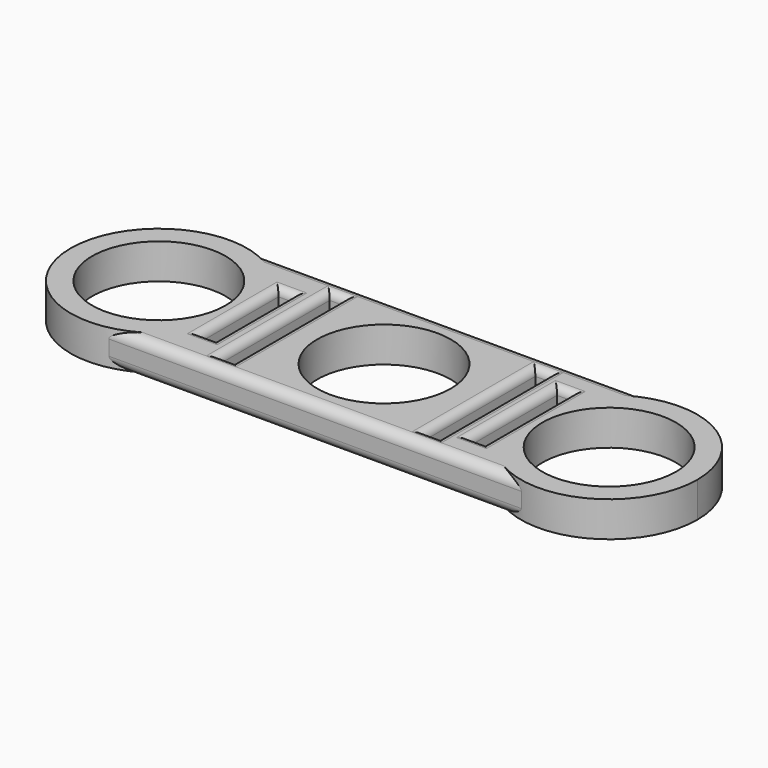
from build123d import *

# Parameters (mm, degrees)
F0_W          = 2.8743222356
F0_H          = 27.3038335145
F0_R          = 13.2535647779
F0_W_2        = 2.8743259609
F1_DEPTH      = 7
F2_R          = 2
F3_T1_DEPTH   = 19.2563887686
F3_T3_DEPTH   = 2.9194724291
F3_T5_DEPTH   = 27.3038335145
F3_T7_DEPTH   = 2.8743222356
F3_T9_DEPTH   = 2.8743259609
F3_T11_DEPTH  = 21.5556565672
F3_T13_DEPTH  = 2.9122043878
F3_T19_DEPTH  = 6.6694724291
F3_T23_DEPTH  = 23.0063887686
F3_T30_DEPTH  = 6.6694724291
F3_T34_DEPTH  = 23.0063887686
F3_T41_DEPTH  = 6.6694724291
F3_T45_DEPTH  = 23.0063887686
F3_T52_DEPTH  = 23.0063887686
F3_T56_DEPTH  = 6.6694724291
F3_T63_DEPTH  = 6.6243222356
F3_T67_DEPTH  = 31.0538335145
F3_T74_DEPTH  = 31.0538335145
F3_T78_DEPTH  = 6.6243222356
F3_T85_DEPTH  = 31.0538335145
F3_T89_DEPTH  = 6.6243222356
F3_T96_DEPTH  = 31.0538335145
F3_T100_DEPTH = 6.6243222356
F3_T107_DEPTH = 6.6243259609
F3_T111_DEPTH = 31.0538335145
F3_T118_DEPTH = 31.0538335145
F3_T122_DEPTH = 6.6243259609
F3_T129_DEPTH = 31.0538335145
F3_T133_DEPTH = 6.6243259609
F3_T140_DEPTH = 31.0538335145
F3_T144_DEPTH = 6.6243259609
F3_T151_DEPTH = 6.6622043878
F3_T155_DEPTH = 25.3056565672
F3_T162_DEPTH = 25.3056565672
F3_T166_DEPTH = 6.6622043878
F3_T173_DEPTH = 6.6622043878
F3_T177_DEPTH = 25.3056565672
F3_T184_DEPTH = 6.6622043878
F3_T188_DEPTH = 25.3056565672
F3_T195_DEPTH = 23.0063887686
F3_T199_DEPTH = 6.6694724291
F3_T206_DEPTH = 6.6694724291
F3_T210_DEPTH = 23.0063887686
F3_T217_DEPTH = 6.6694724291
F3_T221_DEPTH = 23.0063887686
F3_T228_DEPTH = 6.6694724291
F3_T232_DEPTH = 23.0063887686
F3_T239_DEPTH = 31.0538335145
F3_T243_DEPTH = 6.6243222356
F3_T250_DEPTH = 31.0538335145
F3_T254_DEPTH = 6.6243222356
F3_T261_DEPTH = 6.6243222356
F3_T265_DEPTH = 31.0538335145
F3_T272_DEPTH = 31.0538335145
F3_T276_DEPTH = 6.6243222356
F3_T283_DEPTH = 6.6243259609
F3_T287_DEPTH = 31.0538335145
F3_T294_DEPTH = 31.0538335145
F3_T298_DEPTH = 6.6243259609
F3_T305_DEPTH = 31.0538335145
F3_T309_DEPTH = 6.6243259609
F3_T316_DEPTH = 31.0538335145
F3_T320_DEPTH = 6.6243259609
F3_T327_DEPTH = 6.6622043878
F3_T331_DEPTH = 25.3056565672
F3_T338_DEPTH = 6.6622043878
F3_T342_DEPTH = 25.3056565672
F3_T349_DEPTH = 6.6622043878
F3_T353_DEPTH = 25.3056565672
F3_T360_DEPTH = 25.3056565672
F3_T364_DEPTH = 6.6622043878


# Not quite as in the source:
# - a fillet or chamfer that OpenCascade refuses, or shapes differently, is made with other operations: its cross-section is extruded or revolved along the edge and cut away or added


with BuildPart() as f1:
    # F0 (on Top) → F1 (new body)
    with BuildSketch(Plane.XY):
        with BuildLine():
            Line((-40.9337122707, -17.1008221805), (40.9337122707, -17.1008221805))
            ThreePointArc((40.9337122707, -17.1008221805), (33.5711510224, -13.5236311117), (28.6392175138, -6.9906657863))
            Line((28.6392175138, -6.9906657863), (28.6392175138, -10.7778282836))
            Line((28.6392175138, -10.7778282836), (25.727013126, -10.7778282836))
            Line((25.727013126, -10.7778282836), (25.727013126, 10.7778282836))
            Line((25.727013126, 10.7778282836), (28.6392175138, 10.7778282836))
            Line((28.6392175138, 10.7778282836), (28.6392175138, 6.9906657863))
            ThreePointArc((28.6392175138, 6.9906657863), (33.5711510224, 13.5236311117), (40.9337122707, 17.1008221805))
            Line((40.9337122707, 17.1008221805), (-40.9337122707, 17.1008221805))
            ThreePointArc((-40.9337122707, 17.1008221805), (-33.5746643577, 13.5265194749), (-28.6428515345, 6.9990047645))
            Line((-28.6428515345, 6.9990047645), (-28.6428515345, 9.6281943843))
            Line((-28.6428515345, 9.6281943843), (-25.7233791053, 9.6281943843))
            Line((-25.7233791053, 9.6281943843), (-25.7233791053, -9.6281943843))
            Line((-25.7233791053, -9.6281943843), (-28.6428515345, -9.6281943843))
            Line((-28.6428515345, -9.6281943843), (-28.6428515345, -6.9990047645))
            ThreePointArc((-28.6428515345, -6.9990047645), (-33.5746643577, -13.5265194749), (-40.9337122707, -17.1008221805))
        make_face()
        with Locations((-20.2621649951, 0)):
            Rectangle(F0_W, F0_H, mode=Mode.SUBTRACT)
        Circle(F0_R, mode=Mode.SUBTRACT)
        with Locations((20.5532256514, 0)):
            Rectangle(F0_W_2, F0_H, mode=Mode.SUBTRACT)
        with BuildLine():
            ThreePointArc((-40.9337122707, 17.1008221805), (-62.2010158137, 0), (-40.9337122707, -17.1008221805))
            ThreePointArc((-40.9337122707, -17.1008221805), (-33.5746643577, -13.5265194749), (-28.6428515345, -6.9990047645))
            Line((-28.6428515345, -6.9990047645), (-28.6428515345, 6.9990047645))
            ThreePointArc((-28.6428515345, 6.9990047645), (-33.5746643577, 13.5265194749), (-40.9337122707, 17.1008221805))
        make_face()
        with Locations((-44.6920655668, 0)):
            Circle(F0_R, mode=Mode.SUBTRACT)
        with BuildLine():
            ThreePointArc((28.6392175138, -6.9906657863), (33.5711510224, -13.5236311117), (40.9337122707, -17.1008221805))
            ThreePointArc((40.9337122707, -17.1008221805), (55.6638137838, -13.6449287213), (62.2010158137, 0))
            ThreePointArc((62.2010158137, 0), (55.6638137838, 13.6449287213), (40.9337122707, 17.1008221805))
            ThreePointArc((40.9337122707, 17.1008221805), (33.5711510224, 13.5236311117), (28.6392175138, 6.9906657863))
            Line((28.6392175138, 6.9906657863), (28.6392175138, -6.9906657863))
        make_face()
        with Locations((44.6920655668, 0)):
            Circle(F0_R, mode=Mode.SUBTRACT)
    extrude(amount=F1_DEPTH)

    # F2
    f2_edges = [f1.edges().sort_by_distance(p)[0] for p in [
        (0, 17.100822, 7),
        (0, -17.100822, 7),
        (0, -17.100822, 0),
        (0, 17.100822, 0),
    ]]
    fillet(f2_edges, radius=F2_R)

    # F3: fillet of radius 1.5 on 32 edges, made by hand

    # F3_s2 → F3_t1 (cut)
    with BuildSketch(Plane.XZ.offset(-9.6281943843)):
        with BuildLine():
            ThreePointArc((-30.1428515345, 7), (-29.0821913627, 6.5606601718), (-28.6428515345, 5.5))
            Line((-28.6428515345, 5.5), (-28.6428515345, 7))
            Line((-28.6428515345, 7), (-30.1428515345, 7))
        make_face()
        with BuildLine():
            ThreePointArc((-24.2233791053, 7), (-25.2840392771, 6.5606601718), (-25.7233791053, 5.5))
            Line((-25.7233791053, 5.5), (-25.7233791053, 7))
            Line((-25.7233791053, 7), (-24.2233791053, 7))
        make_face()
        with BuildLine():
            ThreePointArc((-30.1428515345, 0), (-29.0821913627, 0.4393398282), (-28.6428515345, 1.5))
            Line((-28.6428515345, 1.5), (-28.6428515345, 0))
            Line((-28.6428515345, 0), (-30.1428515345, 0))
        make_face()
        with BuildLine():
            ThreePointArc((-24.2233791053, 0), (-25.2840392771, 0.4393398282), (-25.7233791053, 1.5))
            Line((-25.7233791053, 1.5), (-25.7233791053, 0))
            Line((-25.7233791053, 0), (-24.2233791053, 0))
        make_face()
    extrude(amount=F3_T1_DEPTH, mode=Mode.SUBTRACT)

    # F3_s4 → F3_t3 (cut)
    with BuildSketch(Plane.YZ.offset(-28.6428515345)):
        with BuildLine():
            ThreePointArc((11.1281943843, 7), (10.0675342125, 6.5606601718), (9.6281943843, 5.5))
            Line((9.6281943843, 5.5), (9.6281943843, 7))
            Line((9.6281943843, 7), (11.1281943843, 7))
        make_face()
        with BuildLine():
            ThreePointArc((-11.1281943843, 7), (-10.0675342125, 6.5606601718), (-9.6281943843, 5.5))
            Line((-9.6281943843, 5.5), (-9.6281943843, 7))
            Line((-9.6281943843, 7), (-11.1281943843, 7))
        make_face()
        with BuildLine():
            ThreePointArc((-11.1281943843, 0), (-10.0675342125, 0.4393398282), (-9.6281943843, 1.5))
            Line((-9.6281943843, 1.5), (-9.6281943843, 0))
            Line((-9.6281943843, 0), (-11.1281943843, 0))
        make_face()
        with BuildLine():
            ThreePointArc((11.1281943843, 0), (10.0675342125, 0.4393398282), (9.6281943843, 1.5))
            Line((9.6281943843, 1.5), (9.6281943843, 0))
            Line((9.6281943843, 0), (11.1281943843, 0))
        make_face()
    extrude(amount=F3_T3_DEPTH, mode=Mode.SUBTRACT)

    # F3_s6 → F3_t5 (cut)
    with BuildSketch(Plane.XZ.offset(-13.6519167572)):
        with BuildLine():
            ThreePointArc((-23.1993261129, 7), (-22.1386659411, 6.5606601718), (-21.6993261129, 5.5))
            Line((-21.6993261129, 5.5), (-21.6993261129, 7))
            Line((-21.6993261129, 7), (-23.1993261129, 7))
        make_face()
        with BuildLine():
            ThreePointArc((-17.3250038773, 7), (-18.3856640491, 6.5606601718), (-18.8250038773, 5.5))
            Line((-18.8250038773, 5.5), (-18.8250038773, 7))
            Line((-18.8250038773, 7), (-17.3250038773, 7))
        make_face()
        with BuildLine():
            ThreePointArc((17.6160626709, 7), (18.6767228427, 6.5606601718), (19.1160626709, 5.5))
            Line((19.1160626709, 5.5), (19.1160626709, 7))
            Line((19.1160626709, 7), (17.6160626709, 7))
        make_face()
        with BuildLine():
            ThreePointArc((23.4903886318, 7), (22.42972846, 6.5606601718), (21.9903886318, 5.5))
            Line((21.9903886318, 5.5), (21.9903886318, 7))
            Line((21.9903886318, 7), (23.4903886318, 7))
        make_face()
        with BuildLine():
            ThreePointArc((-23.1993261129, 0), (-22.1386659411, 0.4393398282), (-21.6993261129, 1.5))
            Line((-21.6993261129, 1.5), (-21.6993261129, 0))
            Line((-21.6993261129, 0), (-23.1993261129, 0))
        make_face()
        with BuildLine():
            ThreePointArc((-17.3250038773, 0), (-18.3856640491, 0.4393398282), (-18.8250038773, 1.5))
            Line((-18.8250038773, 1.5), (-18.8250038773, 0))
            Line((-18.8250038773, 0), (-17.3250038773, 0))
        make_face()
        with BuildLine():
            ThreePointArc((17.6160626709, 0), (18.6767228427, 0.4393398282), (19.1160626709, 1.5))
            Line((19.1160626709, 1.5), (19.1160626709, 0))
            Line((19.1160626709, 0), (17.6160626709, 0))
        make_face()
        with BuildLine():
            ThreePointArc((23.4903886318, 0), (22.42972846, 0.4393398282), (21.9903886318, 1.5))
            Line((21.9903886318, 1.5), (21.9903886318, 0))
            Line((21.9903886318, 0), (23.4903886318, 0))
        make_face()
    extrude(amount=F3_T5_DEPTH, mode=Mode.SUBTRACT)

    # F3_s8 → F3_t7 (cut)
    with BuildSketch(Plane.YZ.offset(-21.6993261129)):
        with BuildLine():
            ThreePointArc((-15.1519167572, 7), (-14.0912565854, 6.5606601718), (-13.6519167572, 5.5))
            Line((-13.6519167572, 5.5), (-13.6519167572, 7))
            Line((-13.6519167572, 7), (-15.1519167572, 7))
        make_face()
        with BuildLine():
            ThreePointArc((15.1519167572, 7), (14.0912565854, 6.5606601718), (13.6519167572, 5.5))
            Line((13.6519167572, 5.5), (13.6519167572, 7))
            Line((13.6519167572, 7), (15.1519167572, 7))
        make_face()
        with BuildLine():
            ThreePointArc((15.1519167572, 0), (14.0912565854, 0.4393398282), (13.6519167572, 1.5))
            Line((13.6519167572, 1.5), (13.6519167572, 0))
            Line((13.6519167572, 0), (15.1519167572, 0))
        make_face()
        with BuildLine():
            ThreePointArc((-15.1519167572, 0), (-14.0912565854, 0.4393398282), (-13.6519167572, 1.5))
            Line((-13.6519167572, 1.5), (-13.6519167572, 0))
            Line((-13.6519167572, 0), (-15.1519167572, 0))
        make_face()
    extrude(amount=F3_T7_DEPTH, mode=Mode.SUBTRACT)

    # F3_s10 → F3_t9 (cut)
    with BuildSketch(Plane.YZ.offset(19.1160626709)):
        with BuildLine():
            ThreePointArc((-15.1519167572, 7), (-14.0912565854, 6.5606601718), (-13.6519167572, 5.5))
            Line((-13.6519167572, 5.5), (-13.6519167572, 7))
            Line((-13.6519167572, 7), (-15.1519167572, 7))
        make_face()
        with BuildLine():
            ThreePointArc((15.1519167572, 7), (14.0912565854, 6.5606601718), (13.6519167572, 5.5))
            Line((13.6519167572, 5.5), (13.6519167572, 7))
            Line((13.6519167572, 7), (15.1519167572, 7))
        make_face()
        with BuildLine():
            ThreePointArc((15.1519167572, 0), (14.0912565854, 0.4393398282), (13.6519167572, 1.5))
            Line((13.6519167572, 1.5), (13.6519167572, 0))
            Line((13.6519167572, 0), (15.1519167572, 0))
        make_face()
        with BuildLine():
            ThreePointArc((-15.1519167572, 0), (-14.0912565854, 0.4393398282), (-13.6519167572, 1.5))
            Line((-13.6519167572, 1.5), (-13.6519167572, 0))
            Line((-13.6519167572, 0), (-15.1519167572, 0))
        make_face()
    extrude(amount=F3_T9_DEPTH, mode=Mode.SUBTRACT)

    # F3_s12 → F3_t11 (cut)
    with BuildSketch(Plane.XZ.offset(-10.7778282836)):
        with BuildLine():
            ThreePointArc((24.227013126, 7), (25.2876732978, 6.5606601718), (25.727013126, 5.5))
            Line((25.727013126, 5.5), (25.727013126, 7))
            Line((25.727013126, 7), (24.227013126, 7))
        make_face()
        with BuildLine():
            ThreePointArc((30.1392175138, 7), (29.078557342, 6.5606601718), (28.6392175138, 5.5))
            Line((28.6392175138, 5.5), (28.6392175138, 7))
            Line((28.6392175138, 7), (30.1392175138, 7))
        make_face()
        with BuildLine():
            ThreePointArc((30.1392175138, 0), (29.078557342, 0.4393398282), (28.6392175138, 1.5))
            Line((28.6392175138, 1.5), (28.6392175138, 0))
            Line((28.6392175138, 0), (30.1392175138, 0))
        make_face()
        with BuildLine():
            ThreePointArc((24.227013126, 0), (25.2876732978, 0.4393398282), (25.727013126, 1.5))
            Line((25.727013126, 1.5), (25.727013126, 0))
            Line((25.727013126, 0), (24.227013126, 0))
        make_face()
    extrude(amount=F3_T11_DEPTH, mode=Mode.SUBTRACT)

    # F3_s14 → F3_t13 (cut)
    with BuildSketch(Plane.YZ.offset(25.727013126)):
        with BuildLine():
            ThreePointArc((12.2778282836, 7), (11.2171681118, 6.5606601718), (10.7778282836, 5.5))
            Line((10.7778282836, 5.5), (10.7778282836, 7))
            Line((10.7778282836, 7), (12.2778282836, 7))
        make_face()
        with BuildLine():
            ThreePointArc((-12.2778282836, 7), (-11.2171681118, 6.5606601718), (-10.7778282836, 5.5))
            Line((-10.7778282836, 5.5), (-10.7778282836, 7))
            Line((-10.7778282836, 7), (-12.2778282836, 7))
        make_face()
        with BuildLine():
            ThreePointArc((-12.2778282836, 0), (-11.2171681118, 0.4393398282), (-10.7778282836, 1.5))
            Line((-10.7778282836, 1.5), (-10.7778282836, 0))
            Line((-10.7778282836, 0), (-12.2778282836, 0))
        make_face()
        with BuildLine():
            ThreePointArc((12.2778282836, 0), (11.2171681118, 0.4393398282), (10.7778282836, 1.5))
            Line((10.7778282836, 1.5), (10.7778282836, 0))
            Line((10.7778282836, 0), (12.2778282836, 0))
        make_face()
    extrude(amount=F3_T13_DEPTH, mode=Mode.SUBTRACT)


with BuildPart() as f3_tool17:
    # F3_s18 → F3_t19 (new body)
    with BuildSketch(Plane.YZ.offset(-25.7233791053)):
        with BuildLine():
            ThreePointArc((-11.1281943843, 7), (-10.0675342125, 6.5606601718), (-9.6281943843, 5.5))
            Line((-9.6281943843, 5.5), (-9.6281943843, 7))
            Line((-9.6281943843, 7), (-11.1281943843, 7))
        make_face()
    extrude(amount=-F3_T19_DEPTH)

    split(bisect_by=Plane.YZ.offset(-28.6428515345), keep=Keep.BOTTOM)


with BuildPart() as f3_tool21:
    # F3_s22 → F3_t23 (new body)
    with BuildSketch(Plane.XZ.offset(13.3781943843)):
        with BuildLine():
            ThreePointArc((-30.1428515345, 7), (-29.0821913627, 6.5606601718), (-28.6428515345, 5.5))
            Line((-28.6428515345, 5.5), (-28.6428515345, 7))
            Line((-28.6428515345, 7), (-30.1428515345, 7))
        make_face()
    extrude(amount=-F3_T23_DEPTH)

    split(bisect_by=Plane.XZ.offset(9.6281943843), keep=Keep.TOP)


with BuildPart() as f3_tool17_1:
    add(f3_tool17.part)

    # F3_t25: intersect F3_tool21
    add(f3_tool21.part, mode=Mode.INTERSECT)


with BuildPart() as f1_1:
    add(f1.part)

    # F3_t15: cut F3_tool17
    add(f3_tool17_1.part, mode=Mode.SUBTRACT)


with BuildPart() as f3_tool28:
    # F3_s29 → F3_t30 (new body)
    with BuildSketch(Plane.YZ.offset(-32.3928515345)):
        with BuildLine():
            ThreePointArc((11.1281943843, 7), (10.0675342125, 6.5606601718), (9.6281943843, 5.5))
            Line((9.6281943843, 5.5), (9.6281943843, 7))
            Line((9.6281943843, 7), (11.1281943843, 7))
        make_face()
    extrude(amount=F3_T30_DEPTH)

    split(bisect_by=Plane.YZ.offset(-28.6428515345), keep=Keep.BOTTOM)


with BuildPart() as f3_tool32:
    # F3_s33 → F3_t34 (new body)
    with BuildSketch(Plane.XZ.offset(9.6281943843)):
        with BuildLine():
            ThreePointArc((-30.1428515345, 7), (-29.0821913627, 6.5606601718), (-28.6428515345, 5.5))
            Line((-28.6428515345, 5.5), (-28.6428515345, 7))
            Line((-28.6428515345, 7), (-30.1428515345, 7))
        make_face()
    extrude(amount=-F3_T34_DEPTH)

    split(bisect_by=Plane.XZ.offset(-9.6281943843), keep=Keep.BOTTOM)


with BuildPart() as f3_tool28_1:
    add(f3_tool28.part)

    # F3_t36: intersect F3_tool32
    add(f3_tool32.part, mode=Mode.INTERSECT)


with BuildPart() as f1_2:
    add(f1_1.part)

    # F3_t26: cut F3_tool28
    add(f3_tool28_1.part, mode=Mode.SUBTRACT)


with BuildPart() as f3_tool39:
    # F3_s40 → F3_t41 (new body)
    with BuildSketch(Plane.YZ.offset(-28.6428515345)):
        with BuildLine():
            ThreePointArc((11.1281943843, 7), (10.0675342125, 6.5606601718), (9.6281943843, 5.5))
            Line((9.6281943843, 5.5), (9.6281943843, 7))
            Line((9.6281943843, 7), (11.1281943843, 7))
        make_face()
    extrude(amount=F3_T41_DEPTH)

    split(bisect_by=Plane.YZ.offset(-25.7233791053), keep=Keep.TOP)


with BuildPart() as f3_tool43:
    # F3_s44 → F3_t45 (new body)
    with BuildSketch(Plane.XZ.offset(-13.3781943843)):
        with BuildLine():
            ThreePointArc((-24.2233791053, 7), (-25.2840392771, 6.5606601718), (-25.7233791053, 5.5))
            Line((-25.7233791053, 5.5), (-25.7233791053, 7))
            Line((-25.7233791053, 7), (-24.2233791053, 7))
        make_face()
    extrude(amount=F3_T45_DEPTH)

    split(bisect_by=Plane.XZ.offset(-9.6281943843), keep=Keep.BOTTOM)


with BuildPart() as f3_tool39_1:
    add(f3_tool39.part)

    # F3_t47: intersect F3_tool43
    add(f3_tool43.part, mode=Mode.INTERSECT)


with BuildPart() as f1_3:
    add(f1_2.part)

    # F3_t37: cut F3_tool39
    add(f3_tool39_1.part, mode=Mode.SUBTRACT)


with BuildPart() as f3_tool50:
    # F3_s51 → F3_t52 (new body)
    with BuildSketch(Plane.XZ.offset(-9.6281943843)):
        with BuildLine():
            ThreePointArc((-24.2233791053, 7), (-25.2840392771, 6.5606601718), (-25.7233791053, 5.5))
            Line((-25.7233791053, 5.5), (-25.7233791053, 7))
            Line((-25.7233791053, 7), (-24.2233791053, 7))
        make_face()
    extrude(amount=F3_T52_DEPTH)

    split(bisect_by=Plane.XZ.offset(9.6281943843), keep=Keep.TOP)


with BuildPart() as f3_tool54:
    # F3_s55 → F3_t56 (new body)
    with BuildSketch(Plane.YZ.offset(-21.9733791053)):
        with BuildLine():
            ThreePointArc((-11.1281943843, 7), (-10.0675342125, 6.5606601718), (-9.6281943843, 5.5))
            Line((-9.6281943843, 5.5), (-9.6281943843, 7))
            Line((-9.6281943843, 7), (-11.1281943843, 7))
        make_face()
    extrude(amount=-F3_T56_DEPTH)

    split(bisect_by=Plane.YZ.offset(-25.7233791053), keep=Keep.TOP)


with BuildPart() as f3_tool50_1:
    add(f3_tool50.part)

    # F3_t58: intersect F3_tool54
    add(f3_tool54.part, mode=Mode.INTERSECT)


with BuildPart() as f1_4:
    add(f1_3.part)

    # F3_t48: cut F3_tool50
    add(f3_tool50_1.part, mode=Mode.SUBTRACT)


with BuildPart() as f3_tool61:
    # F3_s62 → F3_t63 (new body)
    with BuildSketch(Plane.YZ.offset(-18.8250038773)):
        with BuildLine():
            ThreePointArc((-15.1519167572, 7), (-14.0912565854, 6.5606601718), (-13.6519167572, 5.5))
            Line((-13.6519167572, 5.5), (-13.6519167572, 7))
            Line((-13.6519167572, 7), (-15.1519167572, 7))
        make_face()
    extrude(amount=-F3_T63_DEPTH)

    split(bisect_by=Plane.YZ.offset(-21.6993261129), keep=Keep.BOTTOM)


with BuildPart() as f3_tool65:
    # F3_s66 → F3_t67 (new body)
    with BuildSketch(Plane.XZ.offset(17.4019167572)):
        with BuildLine():
            ThreePointArc((-23.1993261129, 7), (-22.1386659411, 6.5606601718), (-21.6993261129, 5.5))
            Line((-21.6993261129, 5.5), (-21.6993261129, 7))
            Line((-21.6993261129, 7), (-23.1993261129, 7))
        make_face()
    extrude(amount=-F3_T67_DEPTH)

    split(bisect_by=Plane.XZ.offset(13.6519167572), keep=Keep.TOP)


with BuildPart() as f3_tool61_1:
    add(f3_tool61.part)

    # F3_t69: intersect F3_tool65
    add(f3_tool65.part, mode=Mode.INTERSECT)


with BuildPart() as f1_5:
    add(f1_4.part)

    # F3_t59: cut F3_tool61
    add(f3_tool61_1.part, mode=Mode.SUBTRACT)


with BuildPart() as f3_tool72:
    # F3_s73 → F3_t74 (new body)
    with BuildSketch(Plane.XZ.offset(13.6519167572)):
        with BuildLine():
            ThreePointArc((-23.1993261129, 7), (-22.1386659411, 6.5606601718), (-21.6993261129, 5.5))
            Line((-21.6993261129, 5.5), (-21.6993261129, 7))
            Line((-21.6993261129, 7), (-23.1993261129, 7))
        make_face()
    extrude(amount=-F3_T74_DEPTH)

    split(bisect_by=Plane.XZ.offset(-13.6519167572), keep=Keep.BOTTOM)


with BuildPart() as f3_tool76:
    # F3_s77 → F3_t78 (new body)
    with BuildSketch(Plane.YZ.offset(-25.4493261129)):
        with BuildLine():
            ThreePointArc((15.1519167572, 7), (14.0912565854, 6.5606601718), (13.6519167572, 5.5))
            Line((13.6519167572, 5.5), (13.6519167572, 7))
            Line((13.6519167572, 7), (15.1519167572, 7))
        make_face()
    extrude(amount=F3_T78_DEPTH)

    split(bisect_by=Plane.YZ.offset(-21.6993261129), keep=Keep.BOTTOM)


with BuildPart() as f3_tool72_1:
    add(f3_tool72.part)

    # F3_t80: intersect F3_tool76
    add(f3_tool76.part, mode=Mode.INTERSECT)


with BuildPart() as f1_6:
    add(f1_5.part)

    # F3_t70: cut F3_tool72
    add(f3_tool72_1.part, mode=Mode.SUBTRACT)


with BuildPart() as f3_tool83:
    # F3_s84 → F3_t85 (new body)
    with BuildSketch(Plane.XZ.offset(-13.6519167572)):
        with BuildLine():
            ThreePointArc((-17.3250038773, 7), (-18.3856640491, 6.5606601718), (-18.8250038773, 5.5))
            Line((-18.8250038773, 5.5), (-18.8250038773, 7))
            Line((-18.8250038773, 7), (-17.3250038773, 7))
        make_face()
    extrude(amount=F3_T85_DEPTH)

    split(bisect_by=Plane.XZ.offset(13.6519167572), keep=Keep.TOP)


with BuildPart() as f3_tool87:
    # F3_s88 → F3_t89 (new body)
    with BuildSketch(Plane.YZ.offset(-15.0750038773)):
        with BuildLine():
            ThreePointArc((-15.1519167572, 7), (-14.0912565854, 6.5606601718), (-13.6519167572, 5.5))
            Line((-13.6519167572, 5.5), (-13.6519167572, 7))
            Line((-13.6519167572, 7), (-15.1519167572, 7))
        make_face()
    extrude(amount=-F3_T89_DEPTH)

    split(bisect_by=Plane.YZ.offset(-18.8250038773), keep=Keep.TOP)


with BuildPart() as f3_tool83_1:
    add(f3_tool83.part)

    # F3_t91: intersect F3_tool87
    add(f3_tool87.part, mode=Mode.INTERSECT)


with BuildPart() as f1_7:
    add(f1_6.part)

    # F3_t81: cut F3_tool83
    add(f3_tool83_1.part, mode=Mode.SUBTRACT)


with BuildPart() as f3_tool94:
    # F3_s95 → F3_t96 (new body)
    with BuildSketch(Plane.XZ.offset(-17.4019167572)):
        with BuildLine():
            ThreePointArc((-17.3250038773, 7), (-18.3856640491, 6.5606601718), (-18.8250038773, 5.5))
            Line((-18.8250038773, 5.5), (-18.8250038773, 7))
            Line((-18.8250038773, 7), (-17.3250038773, 7))
        make_face()
    extrude(amount=F3_T96_DEPTH)

    split(bisect_by=Plane.XZ.offset(-13.6519167572), keep=Keep.BOTTOM)


with BuildPart() as f3_tool98:
    # F3_s99 → F3_t100 (new body)
    with BuildSketch(Plane.YZ.offset(-21.6993261129)):
        with BuildLine():
            ThreePointArc((15.1519167572, 7), (14.0912565854, 6.5606601718), (13.6519167572, 5.5))
            Line((13.6519167572, 5.5), (13.6519167572, 7))
            Line((13.6519167572, 7), (15.1519167572, 7))
        make_face()
    extrude(amount=F3_T100_DEPTH)

    split(bisect_by=Plane.YZ.offset(-18.8250038773), keep=Keep.TOP)


with BuildPart() as f3_tool94_1:
    add(f3_tool94.part)

    # F3_t102: intersect F3_tool98
    add(f3_tool98.part, mode=Mode.INTERSECT)


with BuildPart() as f1_8:
    add(f1_7.part)

    # F3_t92: cut F3_tool94
    add(f3_tool94_1.part, mode=Mode.SUBTRACT)


with BuildPart() as f3_tool105:
    # F3_s106 → F3_t107 (new body)
    with BuildSketch(Plane.YZ.offset(21.9903886318)):
        with BuildLine():
            ThreePointArc((-15.1519167572, 7), (-14.0912565854, 6.5606601718), (-13.6519167572, 5.5))
            Line((-13.6519167572, 5.5), (-13.6519167572, 7))
            Line((-13.6519167572, 7), (-15.1519167572, 7))
        make_face()
    extrude(amount=-F3_T107_DEPTH)

    split(bisect_by=Plane.YZ.offset(19.1160626709), keep=Keep.BOTTOM)


with BuildPart() as f3_tool109:
    # F3_s110 → F3_t111 (new body)
    with BuildSketch(Plane.XZ.offset(17.4019167572)):
        with BuildLine():
            ThreePointArc((17.6160626709, 7), (18.6767228427, 6.5606601718), (19.1160626709, 5.5))
            Line((19.1160626709, 5.5), (19.1160626709, 7))
            Line((19.1160626709, 7), (17.6160626709, 7))
        make_face()
    extrude(amount=-F3_T111_DEPTH)

    split(bisect_by=Plane.XZ.offset(13.6519167572), keep=Keep.TOP)


with BuildPart() as f3_tool105_1:
    add(f3_tool105.part)

    # F3_t113: intersect F3_tool109
    add(f3_tool109.part, mode=Mode.INTERSECT)


with BuildPart() as f1_9:
    add(f1_8.part)

    # F3_t103: cut F3_tool105
    add(f3_tool105_1.part, mode=Mode.SUBTRACT)


with BuildPart() as f3_tool116:
    # F3_s117 → F3_t118 (new body)
    with BuildSketch(Plane.XZ.offset(13.6519167572)):
        with BuildLine():
            ThreePointArc((17.6160626709, 7), (18.6767228427, 6.5606601718), (19.1160626709, 5.5))
            Line((19.1160626709, 5.5), (19.1160626709, 7))
            Line((19.1160626709, 7), (17.6160626709, 7))
        make_face()
    extrude(amount=-F3_T118_DEPTH)

    split(bisect_by=Plane.XZ.offset(-13.6519167572), keep=Keep.BOTTOM)


with BuildPart() as f3_tool120:
    # F3_s121 → F3_t122 (new body)
    with BuildSketch(Plane.YZ.offset(15.3660626709)):
        with BuildLine():
            ThreePointArc((15.1519167572, 7), (14.0912565854, 6.5606601718), (13.6519167572, 5.5))
            Line((13.6519167572, 5.5), (13.6519167572, 7))
            Line((13.6519167572, 7), (15.1519167572, 7))
        make_face()
    extrude(amount=F3_T122_DEPTH)

    split(bisect_by=Plane.YZ.offset(19.1160626709), keep=Keep.BOTTOM)


with BuildPart() as f3_tool116_1:
    add(f3_tool116.part)

    # F3_t124: intersect F3_tool120
    add(f3_tool120.part, mode=Mode.INTERSECT)


with BuildPart() as f1_10:
    add(f1_9.part)

    # F3_t114: cut F3_tool116
    add(f3_tool116_1.part, mode=Mode.SUBTRACT)


with BuildPart() as f3_tool127:
    # F3_s128 → F3_t129 (new body)
    with BuildSketch(Plane.XZ.offset(-17.4019167572)):
        with BuildLine():
            ThreePointArc((23.4903886318, 7), (22.42972846, 6.5606601718), (21.9903886318, 5.5))
            Line((21.9903886318, 5.5), (21.9903886318, 7))
            Line((21.9903886318, 7), (23.4903886318, 7))
        make_face()
    extrude(amount=F3_T129_DEPTH)

    split(bisect_by=Plane.XZ.offset(-13.6519167572), keep=Keep.BOTTOM)


with BuildPart() as f3_tool131:
    # F3_s132 → F3_t133 (new body)
    with BuildSketch(Plane.YZ.offset(19.1160626709)):
        with BuildLine():
            ThreePointArc((15.1519167572, 7), (14.0912565854, 6.5606601718), (13.6519167572, 5.5))
            Line((13.6519167572, 5.5), (13.6519167572, 7))
            Line((13.6519167572, 7), (15.1519167572, 7))
        make_face()
    extrude(amount=F3_T133_DEPTH)

    split(bisect_by=Plane.YZ.offset(21.9903886318), keep=Keep.TOP)


with BuildPart() as f3_tool127_1:
    add(f3_tool127.part)

    # F3_t135: intersect F3_tool131
    add(f3_tool131.part, mode=Mode.INTERSECT)


with BuildPart() as f1_11:
    add(f1_10.part)

    # F3_t125: cut F3_tool127
    add(f3_tool127_1.part, mode=Mode.SUBTRACT)


with BuildPart() as f3_tool138:
    # F3_s139 → F3_t140 (new body)
    with BuildSketch(Plane.XZ.offset(-13.6519167572)):
        with BuildLine():
            ThreePointArc((23.4903886318, 7), (22.42972846, 6.5606601718), (21.9903886318, 5.5))
            Line((21.9903886318, 5.5), (21.9903886318, 7))
            Line((21.9903886318, 7), (23.4903886318, 7))
        make_face()
    extrude(amount=F3_T140_DEPTH)

    split(bisect_by=Plane.XZ.offset(13.6519167572), keep=Keep.TOP)


with BuildPart() as f3_tool142:
    # F3_s143 → F3_t144 (new body)
    with BuildSketch(Plane.YZ.offset(25.7403886318)):
        with BuildLine():
            ThreePointArc((-15.1519167572, 7), (-14.0912565854, 6.5606601718), (-13.6519167572, 5.5))
            Line((-13.6519167572, 5.5), (-13.6519167572, 7))
            Line((-13.6519167572, 7), (-15.1519167572, 7))
        make_face()
    extrude(amount=-F3_T144_DEPTH)

    split(bisect_by=Plane.YZ.offset(21.9903886318), keep=Keep.TOP)


with BuildPart() as f3_tool138_1:
    add(f3_tool138.part)

    # F3_t146: intersect F3_tool142
    add(f3_tool142.part, mode=Mode.INTERSECT)


with BuildPart() as f1_12:
    add(f1_11.part)

    # F3_t136: cut F3_tool138
    add(f3_tool138_1.part, mode=Mode.SUBTRACT)


with BuildPart() as f3_tool149:
    # F3_s150 → F3_t151 (new body)
    with BuildSketch(Plane.YZ.offset(28.6392175138)):
        with BuildLine():
            ThreePointArc((-12.2778282836, 7), (-11.2171681118, 6.5606601718), (-10.7778282836, 5.5))
            Line((-10.7778282836, 5.5), (-10.7778282836, 7))
            Line((-10.7778282836, 7), (-12.2778282836, 7))
        make_face()
    extrude(amount=-F3_T151_DEPTH)

    split(bisect_by=Plane.YZ.offset(25.727013126), keep=Keep.BOTTOM)


with BuildPart() as f3_tool153:
    # F3_s154 → F3_t155 (new body)
    with BuildSketch(Plane.XZ.offset(14.5278282836)):
        with BuildLine():
            ThreePointArc((24.227013126, 7), (25.2876732978, 6.5606601718), (25.727013126, 5.5))
            Line((25.727013126, 5.5), (25.727013126, 7))
            Line((25.727013126, 7), (24.227013126, 7))
        make_face()
    extrude(amount=-F3_T155_DEPTH)

    split(bisect_by=Plane.XZ.offset(10.7778282836), keep=Keep.TOP)


with BuildPart() as f3_tool149_1:
    add(f3_tool149.part)

    # F3_t157: intersect F3_tool153
    add(f3_tool153.part, mode=Mode.INTERSECT)


with BuildPart() as f1_13:
    add(f1_12.part)

    # F3_t147: cut F3_tool149
    add(f3_tool149_1.part, mode=Mode.SUBTRACT)


with BuildPart() as f3_tool160:
    # F3_s161 → F3_t162 (new body)
    with BuildSketch(Plane.XZ.offset(10.7778282836)):
        with BuildLine():
            ThreePointArc((24.227013126, 7), (25.2876732978, 6.5606601718), (25.727013126, 5.5))
            Line((25.727013126, 5.5), (25.727013126, 7))
            Line((25.727013126, 7), (24.227013126, 7))
        make_face()
    extrude(amount=-F3_T162_DEPTH)

    split(bisect_by=Plane.XZ.offset(-10.7778282836), keep=Keep.BOTTOM)


with BuildPart() as f3_tool164:
    # F3_s165 → F3_t166 (new body)
    with BuildSketch(Plane.YZ.offset(21.977013126)):
        with BuildLine():
            ThreePointArc((12.2778282836, 7), (11.2171681118, 6.5606601718), (10.7778282836, 5.5))
            Line((10.7778282836, 5.5), (10.7778282836, 7))
            Line((10.7778282836, 7), (12.2778282836, 7))
        make_face()
    extrude(amount=F3_T166_DEPTH)

    split(bisect_by=Plane.YZ.offset(25.727013126), keep=Keep.BOTTOM)


with BuildPart() as f3_tool160_1:
    add(f3_tool160.part)

    # F3_t168: intersect F3_tool164
    add(f3_tool164.part, mode=Mode.INTERSECT)


with BuildPart() as f1_14:
    add(f1_13.part)

    # F3_t158: cut F3_tool160
    add(f3_tool160_1.part, mode=Mode.SUBTRACT)


with BuildPart() as f3_tool171:
    # F3_s172 → F3_t173 (new body)
    with BuildSketch(Plane.YZ.offset(25.727013126)):
        with BuildLine():
            ThreePointArc((12.2778282836, 7), (11.2171681118, 6.5606601718), (10.7778282836, 5.5))
            Line((10.7778282836, 5.5), (10.7778282836, 7))
            Line((10.7778282836, 7), (12.2778282836, 7))
        make_face()
    extrude(amount=F3_T173_DEPTH)

    split(bisect_by=Plane.YZ.offset(28.6392175138), keep=Keep.TOP)


with BuildPart() as f3_tool175:
    # F3_s176 → F3_t177 (new body)
    with BuildSketch(Plane.XZ.offset(-14.5278282836)):
        with BuildLine():
            ThreePointArc((30.1392175138, 7), (29.078557342, 6.5606601718), (28.6392175138, 5.5))
            Line((28.6392175138, 5.5), (28.6392175138, 7))
            Line((28.6392175138, 7), (30.1392175138, 7))
        make_face()
    extrude(amount=F3_T177_DEPTH)

    split(bisect_by=Plane.XZ.offset(-10.7778282836), keep=Keep.BOTTOM)


with BuildPart() as f3_tool171_1:
    add(f3_tool171.part)

    # F3_t179: intersect F3_tool175
    add(f3_tool175.part, mode=Mode.INTERSECT)


with BuildPart() as f1_15:
    add(f1_14.part)

    # F3_t169: cut F3_tool171
    add(f3_tool171_1.part, mode=Mode.SUBTRACT)


with BuildPart() as f3_tool182:
    # F3_s183 → F3_t184 (new body)
    with BuildSketch(Plane.YZ.offset(32.3892175138)):
        with BuildLine():
            ThreePointArc((-12.2778282836, 7), (-11.2171681118, 6.5606601718), (-10.7778282836, 5.5))
            Line((-10.7778282836, 5.5), (-10.7778282836, 7))
            Line((-10.7778282836, 7), (-12.2778282836, 7))
        make_face()
    extrude(amount=-F3_T184_DEPTH)

    split(bisect_by=Plane.YZ.offset(28.6392175138), keep=Keep.TOP)


with BuildPart() as f3_tool186:
    # F3_s187 → F3_t188 (new body)
    with BuildSketch(Plane.XZ.offset(-10.7778282836)):
        with BuildLine():
            ThreePointArc((30.1392175138, 7), (29.078557342, 6.5606601718), (28.6392175138, 5.5))
            Line((28.6392175138, 5.5), (28.6392175138, 7))
            Line((28.6392175138, 7), (30.1392175138, 7))
        make_face()
    extrude(amount=F3_T188_DEPTH)

    split(bisect_by=Plane.XZ.offset(10.7778282836), keep=Keep.TOP)


with BuildPart() as f3_tool182_1:
    add(f3_tool182.part)

    # F3_t190: intersect F3_tool186
    add(f3_tool186.part, mode=Mode.INTERSECT)


with BuildPart() as f1_16:
    add(f1_15.part)

    # F3_t180: cut F3_tool182
    add(f3_tool182_1.part, mode=Mode.SUBTRACT)


with BuildPart() as f3_tool193:
    # F3_s194 → F3_t195 (new body)
    with BuildSketch(Plane.XZ.offset(-9.6281943843)):
        with BuildLine():
            ThreePointArc((-24.2233791053, 0), (-25.2840392771, 0.4393398282), (-25.7233791053, 1.5))
            Line((-25.7233791053, 1.5), (-25.7233791053, 0))
            Line((-25.7233791053, 0), (-24.2233791053, 0))
        make_face()
    extrude(amount=F3_T195_DEPTH)

    split(bisect_by=Plane.XZ.offset(9.6281943843), keep=Keep.TOP)


with BuildPart() as f3_tool197:
    # F3_s198 → F3_t199 (new body)
    with BuildSketch(Plane.YZ.offset(-21.9733791053)):
        with BuildLine():
            ThreePointArc((-11.1281943843, 0), (-10.0675342125, 0.4393398282), (-9.6281943843, 1.5))
            Line((-9.6281943843, 1.5), (-9.6281943843, 0))
            Line((-9.6281943843, 0), (-11.1281943843, 0))
        make_face()
    extrude(amount=-F3_T199_DEPTH)

    split(bisect_by=Plane.YZ.offset(-25.7233791053), keep=Keep.TOP)


with BuildPart() as f3_tool193_1:
    add(f3_tool193.part)

    # F3_t201: intersect F3_tool197
    add(f3_tool197.part, mode=Mode.INTERSECT)


with BuildPart() as f1_17:
    add(f1_16.part)

    # F3_t191: cut F3_tool193
    add(f3_tool193_1.part, mode=Mode.SUBTRACT)


with BuildPart() as f3_tool204:
    # F3_s205 → F3_t206 (new body)
    with BuildSketch(Plane.YZ.offset(-25.7233791053)):
        with BuildLine():
            ThreePointArc((-11.1281943843, 0), (-10.0675342125, 0.4393398282), (-9.6281943843, 1.5))
            Line((-9.6281943843, 1.5), (-9.6281943843, 0))
            Line((-9.6281943843, 0), (-11.1281943843, 0))
        make_face()
    extrude(amount=-F3_T206_DEPTH)

    split(bisect_by=Plane.YZ.offset(-28.6428515345), keep=Keep.BOTTOM)


with BuildPart() as f3_tool208:
    # F3_s209 → F3_t210 (new body)
    with BuildSketch(Plane.XZ.offset(13.3781943843)):
        with BuildLine():
            ThreePointArc((-30.1428515345, 0), (-29.0821913627, 0.4393398282), (-28.6428515345, 1.5))
            Line((-28.6428515345, 1.5), (-28.6428515345, 0))
            Line((-28.6428515345, 0), (-30.1428515345, 0))
        make_face()
    extrude(amount=-F3_T210_DEPTH)

    split(bisect_by=Plane.XZ.offset(9.6281943843), keep=Keep.TOP)


with BuildPart() as f3_tool204_1:
    add(f3_tool204.part)

    # F3_t212: intersect F3_tool208
    add(f3_tool208.part, mode=Mode.INTERSECT)


with BuildPart() as f1_18:
    add(f1_17.part)

    # F3_t202: cut F3_tool204
    add(f3_tool204_1.part, mode=Mode.SUBTRACT)


with BuildPart() as f3_tool215:
    # F3_s216 → F3_t217 (new body)
    with BuildSketch(Plane.YZ.offset(-32.3928515345)):
        with BuildLine():
            ThreePointArc((11.1281943843, 0), (10.0675342125, 0.4393398282), (9.6281943843, 1.5))
            Line((9.6281943843, 1.5), (9.6281943843, 0))
            Line((9.6281943843, 0), (11.1281943843, 0))
        make_face()
    extrude(amount=F3_T217_DEPTH)

    split(bisect_by=Plane.YZ.offset(-28.6428515345), keep=Keep.BOTTOM)


with BuildPart() as f3_tool219:
    # F3_s220 → F3_t221 (new body)
    with BuildSketch(Plane.XZ.offset(9.6281943843)):
        with BuildLine():
            ThreePointArc((-30.1428515345, 0), (-29.0821913627, 0.4393398282), (-28.6428515345, 1.5))
            Line((-28.6428515345, 1.5), (-28.6428515345, 0))
            Line((-28.6428515345, 0), (-30.1428515345, 0))
        make_face()
    extrude(amount=-F3_T221_DEPTH)

    split(bisect_by=Plane.XZ.offset(-9.6281943843), keep=Keep.BOTTOM)


with BuildPart() as f3_tool215_1:
    add(f3_tool215.part)

    # F3_t223: intersect F3_tool219
    add(f3_tool219.part, mode=Mode.INTERSECT)


with BuildPart() as f1_19:
    add(f1_18.part)

    # F3_t213: cut F3_tool215
    add(f3_tool215_1.part, mode=Mode.SUBTRACT)


with BuildPart() as f3_tool226:
    # F3_s227 → F3_t228 (new body)
    with BuildSketch(Plane.YZ.offset(-28.6428515345)):
        with BuildLine():
            ThreePointArc((11.1281943843, 0), (10.0675342125, 0.4393398282), (9.6281943843, 1.5))
            Line((9.6281943843, 1.5), (9.6281943843, 0))
            Line((9.6281943843, 0), (11.1281943843, 0))
        make_face()
    extrude(amount=F3_T228_DEPTH)

    split(bisect_by=Plane.YZ.offset(-25.7233791053), keep=Keep.TOP)


with BuildPart() as f3_tool230:
    # F3_s231 → F3_t232 (new body)
    with BuildSketch(Plane.XZ.offset(-13.3781943843)):
        with BuildLine():
            ThreePointArc((-24.2233791053, 0), (-25.2840392771, 0.4393398282), (-25.7233791053, 1.5))
            Line((-25.7233791053, 1.5), (-25.7233791053, 0))
            Line((-25.7233791053, 0), (-24.2233791053, 0))
        make_face()
    extrude(amount=F3_T232_DEPTH)

    split(bisect_by=Plane.XZ.offset(-9.6281943843), keep=Keep.BOTTOM)


with BuildPart() as f3_tool226_1:
    add(f3_tool226.part)

    # F3_t234: intersect F3_tool230
    add(f3_tool230.part, mode=Mode.INTERSECT)


with BuildPart() as f1_20:
    add(f1_19.part)

    # F3_t224: cut F3_tool226
    add(f3_tool226_1.part, mode=Mode.SUBTRACT)


with BuildPart() as f3_tool237:
    # F3_s238 → F3_t239 (new body)
    with BuildSketch(Plane.XZ.offset(13.6519167572)):
        with BuildLine():
            ThreePointArc((-23.1993261129, 0), (-22.1386659411, 0.4393398282), (-21.6993261129, 1.5))
            Line((-21.6993261129, 1.5), (-21.6993261129, 0))
            Line((-21.6993261129, 0), (-23.1993261129, 0))
        make_face()
    extrude(amount=-F3_T239_DEPTH)

    split(bisect_by=Plane.XZ.offset(-13.6519167572), keep=Keep.BOTTOM)


with BuildPart() as f3_tool241:
    # F3_s242 → F3_t243 (new body)
    with BuildSketch(Plane.YZ.offset(-25.4493261129)):
        with BuildLine():
            ThreePointArc((15.1519167572, 0), (14.0912565854, 0.4393398282), (13.6519167572, 1.5))
            Line((13.6519167572, 1.5), (13.6519167572, 0))
            Line((13.6519167572, 0), (15.1519167572, 0))
        make_face()
    extrude(amount=F3_T243_DEPTH)

    split(bisect_by=Plane.YZ.offset(-21.6993261129), keep=Keep.BOTTOM)


with BuildPart() as f3_tool237_1:
    add(f3_tool237.part)

    # F3_t245: intersect F3_tool241
    add(f3_tool241.part, mode=Mode.INTERSECT)


with BuildPart() as f1_21:
    add(f1_20.part)

    # F3_t235: cut F3_tool237
    add(f3_tool237_1.part, mode=Mode.SUBTRACT)


with BuildPart() as f3_tool248:
    # F3_s249 → F3_t250 (new body)
    with BuildSketch(Plane.XZ.offset(-17.4019167572)):
        with BuildLine():
            ThreePointArc((-17.3250038773, 0), (-18.3856640491, 0.4393398282), (-18.8250038773, 1.5))
            Line((-18.8250038773, 1.5), (-18.8250038773, 0))
            Line((-18.8250038773, 0), (-17.3250038773, 0))
        make_face()
    extrude(amount=F3_T250_DEPTH)

    split(bisect_by=Plane.XZ.offset(-13.6519167572), keep=Keep.BOTTOM)


with BuildPart() as f3_tool252:
    # F3_s253 → F3_t254 (new body)
    with BuildSketch(Plane.YZ.offset(-21.6993261129)):
        with BuildLine():
            ThreePointArc((15.1519167572, 0), (14.0912565854, 0.4393398282), (13.6519167572, 1.5))
            Line((13.6519167572, 1.5), (13.6519167572, 0))
            Line((13.6519167572, 0), (15.1519167572, 0))
        make_face()
    extrude(amount=F3_T254_DEPTH)

    split(bisect_by=Plane.YZ.offset(-18.8250038773), keep=Keep.TOP)


with BuildPart() as f3_tool248_1:
    add(f3_tool248.part)

    # F3_t256: intersect F3_tool252
    add(f3_tool252.part, mode=Mode.INTERSECT)


with BuildPart() as f1_22:
    add(f1_21.part)

    # F3_t246: cut F3_tool248
    add(f3_tool248_1.part, mode=Mode.SUBTRACT)


with BuildPart() as f3_tool259:
    # F3_s260 → F3_t261 (new body)
    with BuildSketch(Plane.YZ.offset(-18.8250038773)):
        with BuildLine():
            ThreePointArc((-15.1519167572, 0), (-14.0912565854, 0.4393398282), (-13.6519167572, 1.5))
            Line((-13.6519167572, 1.5), (-13.6519167572, 0))
            Line((-13.6519167572, 0), (-15.1519167572, 0))
        make_face()
    extrude(amount=-F3_T261_DEPTH)

    split(bisect_by=Plane.YZ.offset(-21.6993261129), keep=Keep.BOTTOM)


with BuildPart() as f3_tool263:
    # F3_s264 → F3_t265 (new body)
    with BuildSketch(Plane.XZ.offset(17.4019167572)):
        with BuildLine():
            ThreePointArc((-23.1993261129, 0), (-22.1386659411, 0.4393398282), (-21.6993261129, 1.5))
            Line((-21.6993261129, 1.5), (-21.6993261129, 0))
            Line((-21.6993261129, 0), (-23.1993261129, 0))
        make_face()
    extrude(amount=-F3_T265_DEPTH)

    split(bisect_by=Plane.XZ.offset(13.6519167572), keep=Keep.TOP)


with BuildPart() as f3_tool259_1:
    add(f3_tool259.part)

    # F3_t267: intersect F3_tool263
    add(f3_tool263.part, mode=Mode.INTERSECT)


with BuildPart() as f1_23:
    add(f1_22.part)

    # F3_t257: cut F3_tool259
    add(f3_tool259_1.part, mode=Mode.SUBTRACT)


with BuildPart() as f3_tool270:
    # F3_s271 → F3_t272 (new body)
    with BuildSketch(Plane.XZ.offset(-13.6519167572)):
        with BuildLine():
            ThreePointArc((-17.3250038773, 0), (-18.3856640491, 0.4393398282), (-18.8250038773, 1.5))
            Line((-18.8250038773, 1.5), (-18.8250038773, 0))
            Line((-18.8250038773, 0), (-17.3250038773, 0))
        make_face()
    extrude(amount=F3_T272_DEPTH)

    split(bisect_by=Plane.XZ.offset(13.6519167572), keep=Keep.TOP)


with BuildPart() as f3_tool274:
    # F3_s275 → F3_t276 (new body)
    with BuildSketch(Plane.YZ.offset(-15.0750038773)):
        with BuildLine():
            ThreePointArc((-15.1519167572, 0), (-14.0912565854, 0.4393398282), (-13.6519167572, 1.5))
            Line((-13.6519167572, 1.5), (-13.6519167572, 0))
            Line((-13.6519167572, 0), (-15.1519167572, 0))
        make_face()
    extrude(amount=-F3_T276_DEPTH)

    split(bisect_by=Plane.YZ.offset(-18.8250038773), keep=Keep.TOP)


with BuildPart() as f3_tool270_1:
    add(f3_tool270.part)

    # F3_t278: intersect F3_tool274
    add(f3_tool274.part, mode=Mode.INTERSECT)


with BuildPart() as f1_24:
    add(f1_23.part)

    # F3_t268: cut F3_tool270
    add(f3_tool270_1.part, mode=Mode.SUBTRACT)


with BuildPart() as f3_tool281:
    # F3_s282 → F3_t283 (new body)
    with BuildSketch(Plane.YZ.offset(21.9903886318)):
        with BuildLine():
            ThreePointArc((-15.1519167572, 0), (-14.0912565854, 0.4393398282), (-13.6519167572, 1.5))
            Line((-13.6519167572, 1.5), (-13.6519167572, 0))
            Line((-13.6519167572, 0), (-15.1519167572, 0))
        make_face()
    extrude(amount=-F3_T283_DEPTH)

    split(bisect_by=Plane.YZ.offset(19.1160626709), keep=Keep.BOTTOM)


with BuildPart() as f3_tool285:
    # F3_s286 → F3_t287 (new body)
    with BuildSketch(Plane.XZ.offset(17.4019167572)):
        with BuildLine():
            ThreePointArc((17.6160626709, 0), (18.6767228427, 0.4393398282), (19.1160626709, 1.5))
            Line((19.1160626709, 1.5), (19.1160626709, 0))
            Line((19.1160626709, 0), (17.6160626709, 0))
        make_face()
    extrude(amount=-F3_T287_DEPTH)

    split(bisect_by=Plane.XZ.offset(13.6519167572), keep=Keep.TOP)


with BuildPart() as f3_tool281_1:
    add(f3_tool281.part)

    # F3_t289: intersect F3_tool285
    add(f3_tool285.part, mode=Mode.INTERSECT)


with BuildPart() as f1_25:
    add(f1_24.part)

    # F3_t279: cut F3_tool281
    add(f3_tool281_1.part, mode=Mode.SUBTRACT)


with BuildPart() as f3_tool292:
    # F3_s293 → F3_t294 (new body)
    with BuildSketch(Plane.XZ.offset(13.6519167572)):
        with BuildLine():
            ThreePointArc((17.6160626709, 0), (18.6767228427, 0.4393398282), (19.1160626709, 1.5))
            Line((19.1160626709, 1.5), (19.1160626709, 0))
            Line((19.1160626709, 0), (17.6160626709, 0))
        make_face()
    extrude(amount=-F3_T294_DEPTH)

    split(bisect_by=Plane.XZ.offset(-13.6519167572), keep=Keep.BOTTOM)


with BuildPart() as f3_tool296:
    # F3_s297 → F3_t298 (new body)
    with BuildSketch(Plane.YZ.offset(15.3660626709)):
        with BuildLine():
            ThreePointArc((15.1519167572, 0), (14.0912565854, 0.4393398282), (13.6519167572, 1.5))
            Line((13.6519167572, 1.5), (13.6519167572, 0))
            Line((13.6519167572, 0), (15.1519167572, 0))
        make_face()
    extrude(amount=F3_T298_DEPTH)

    split(bisect_by=Plane.YZ.offset(19.1160626709), keep=Keep.BOTTOM)


with BuildPart() as f3_tool292_1:
    add(f3_tool292.part)

    # F3_t300: intersect F3_tool296
    add(f3_tool296.part, mode=Mode.INTERSECT)


with BuildPart() as f1_26:
    add(f1_25.part)

    # F3_t290: cut F3_tool292
    add(f3_tool292_1.part, mode=Mode.SUBTRACT)


with BuildPart() as f3_tool303:
    # F3_s304 → F3_t305 (new body)
    with BuildSketch(Plane.XZ.offset(-17.4019167572)):
        with BuildLine():
            ThreePointArc((23.4903886318, 0), (22.42972846, 0.4393398282), (21.9903886318, 1.5))
            Line((21.9903886318, 1.5), (21.9903886318, 0))
            Line((21.9903886318, 0), (23.4903886318, 0))
        make_face()
    extrude(amount=F3_T305_DEPTH)

    split(bisect_by=Plane.XZ.offset(-13.6519167572), keep=Keep.BOTTOM)


with BuildPart() as f3_tool307:
    # F3_s308 → F3_t309 (new body)
    with BuildSketch(Plane.YZ.offset(19.1160626709)):
        with BuildLine():
            ThreePointArc((15.1519167572, 0), (14.0912565854, 0.4393398282), (13.6519167572, 1.5))
            Line((13.6519167572, 1.5), (13.6519167572, 0))
            Line((13.6519167572, 0), (15.1519167572, 0))
        make_face()
    extrude(amount=F3_T309_DEPTH)

    split(bisect_by=Plane.YZ.offset(21.9903886318), keep=Keep.TOP)


with BuildPart() as f3_tool303_1:
    add(f3_tool303.part)

    # F3_t311: intersect F3_tool307
    add(f3_tool307.part, mode=Mode.INTERSECT)


with BuildPart() as f1_27:
    add(f1_26.part)

    # F3_t301: cut F3_tool303
    add(f3_tool303_1.part, mode=Mode.SUBTRACT)


with BuildPart() as f3_tool314:
    # F3_s315 → F3_t316 (new body)
    with BuildSketch(Plane.XZ.offset(-13.6519167572)):
        with BuildLine():
            ThreePointArc((23.4903886318, 0), (22.42972846, 0.4393398282), (21.9903886318, 1.5))
            Line((21.9903886318, 1.5), (21.9903886318, 0))
            Line((21.9903886318, 0), (23.4903886318, 0))
        make_face()
    extrude(amount=F3_T316_DEPTH)

    split(bisect_by=Plane.XZ.offset(13.6519167572), keep=Keep.TOP)


with BuildPart() as f3_tool318:
    # F3_s319 → F3_t320 (new body)
    with BuildSketch(Plane.YZ.offset(25.7403886318)):
        with BuildLine():
            ThreePointArc((-15.1519167572, 0), (-14.0912565854, 0.4393398282), (-13.6519167572, 1.5))
            Line((-13.6519167572, 1.5), (-13.6519167572, 0))
            Line((-13.6519167572, 0), (-15.1519167572, 0))
        make_face()
    extrude(amount=-F3_T320_DEPTH)

    split(bisect_by=Plane.YZ.offset(21.9903886318), keep=Keep.TOP)


with BuildPart() as f3_tool314_1:
    add(f3_tool314.part)

    # F3_t322: intersect F3_tool318
    add(f3_tool318.part, mode=Mode.INTERSECT)


with BuildPart() as f1_28:
    add(f1_27.part)

    # F3_t312: cut F3_tool314
    add(f3_tool314_1.part, mode=Mode.SUBTRACT)


with BuildPart() as f3_tool325:
    # F3_s326 → F3_t327 (new body)
    with BuildSketch(Plane.YZ.offset(32.3892175138)):
        with BuildLine():
            ThreePointArc((-12.2778282836, 0), (-11.2171681118, 0.4393398282), (-10.7778282836, 1.5))
            Line((-10.7778282836, 1.5), (-10.7778282836, 0))
            Line((-10.7778282836, 0), (-12.2778282836, 0))
        make_face()
    extrude(amount=-F3_T327_DEPTH)

    split(bisect_by=Plane.YZ.offset(28.6392175138), keep=Keep.TOP)


with BuildPart() as f3_tool329:
    # F3_s330 → F3_t331 (new body)
    with BuildSketch(Plane.XZ.offset(-10.7778282836)):
        with BuildLine():
            ThreePointArc((30.1392175138, 0), (29.078557342, 0.4393398282), (28.6392175138, 1.5))
            Line((28.6392175138, 1.5), (28.6392175138, 0))
            Line((28.6392175138, 0), (30.1392175138, 0))
        make_face()
    extrude(amount=F3_T331_DEPTH)

    split(bisect_by=Plane.XZ.offset(10.7778282836), keep=Keep.TOP)


with BuildPart() as f3_tool325_1:
    add(f3_tool325.part)

    # F3_t333: intersect F3_tool329
    add(f3_tool329.part, mode=Mode.INTERSECT)


with BuildPart() as f1_29:
    add(f1_28.part)

    # F3_t323: cut F3_tool325
    add(f3_tool325_1.part, mode=Mode.SUBTRACT)


with BuildPart() as f3_tool336:
    # F3_s337 → F3_t338 (new body)
    with BuildSketch(Plane.YZ.offset(28.6392175138)):
        with BuildLine():
            ThreePointArc((-12.2778282836, 0), (-11.2171681118, 0.4393398282), (-10.7778282836, 1.5))
            Line((-10.7778282836, 1.5), (-10.7778282836, 0))
            Line((-10.7778282836, 0), (-12.2778282836, 0))
        make_face()
    extrude(amount=-F3_T338_DEPTH)

    split(bisect_by=Plane.YZ.offset(25.727013126), keep=Keep.BOTTOM)


with BuildPart() as f3_tool340:
    # F3_s341 → F3_t342 (new body)
    with BuildSketch(Plane.XZ.offset(14.5278282836)):
        with BuildLine():
            ThreePointArc((24.227013126, 0), (25.2876732978, 0.4393398282), (25.727013126, 1.5))
            Line((25.727013126, 1.5), (25.727013126, 0))
            Line((25.727013126, 0), (24.227013126, 0))
        make_face()
    extrude(amount=-F3_T342_DEPTH)

    split(bisect_by=Plane.XZ.offset(10.7778282836), keep=Keep.TOP)


with BuildPart() as f3_tool336_1:
    add(f3_tool336.part)

    # F3_t344: intersect F3_tool340
    add(f3_tool340.part, mode=Mode.INTERSECT)


with BuildPart() as f1_30:
    add(f1_29.part)

    # F3_t334: cut F3_tool336
    add(f3_tool336_1.part, mode=Mode.SUBTRACT)


with BuildPart() as f3_tool347:
    # F3_s348 → F3_t349 (new body)
    with BuildSketch(Plane.YZ.offset(25.727013126)):
        with BuildLine():
            ThreePointArc((12.2778282836, 0), (11.2171681118, 0.4393398282), (10.7778282836, 1.5))
            Line((10.7778282836, 1.5), (10.7778282836, 0))
            Line((10.7778282836, 0), (12.2778282836, 0))
        make_face()
    extrude(amount=F3_T349_DEPTH)

    split(bisect_by=Plane.YZ.offset(28.6392175138), keep=Keep.TOP)


with BuildPart() as f3_tool351:
    # F3_s352 → F3_t353 (new body)
    with BuildSketch(Plane.XZ.offset(-14.5278282836)):
        with BuildLine():
            ThreePointArc((30.1392175138, 0), (29.078557342, 0.4393398282), (28.6392175138, 1.5))
            Line((28.6392175138, 1.5), (28.6392175138, 0))
            Line((28.6392175138, 0), (30.1392175138, 0))
        make_face()
    extrude(amount=F3_T353_DEPTH)

    split(bisect_by=Plane.XZ.offset(-10.7778282836), keep=Keep.BOTTOM)


with BuildPart() as f3_tool347_1:
    add(f3_tool347.part)

    # F3_t355: intersect F3_tool351
    add(f3_tool351.part, mode=Mode.INTERSECT)


with BuildPart() as f1_31:
    add(f1_30.part)

    # F3_t345: cut F3_tool347
    add(f3_tool347_1.part, mode=Mode.SUBTRACT)


with BuildPart() as f3_tool358:
    # F3_s359 → F3_t360 (new body)
    with BuildSketch(Plane.XZ.offset(10.7778282836)):
        with BuildLine():
            ThreePointArc((24.227013126, 0), (25.2876732978, 0.4393398282), (25.727013126, 1.5))
            Line((25.727013126, 1.5), (25.727013126, 0))
            Line((25.727013126, 0), (24.227013126, 0))
        make_face()
    extrude(amount=-F3_T360_DEPTH)

    split(bisect_by=Plane.XZ.offset(-10.7778282836), keep=Keep.BOTTOM)


with BuildPart() as f3_tool362:
    # F3_s363 → F3_t364 (new body)
    with BuildSketch(Plane.YZ.offset(21.977013126)):
        with BuildLine():
            ThreePointArc((12.2778282836, 0), (11.2171681118, 0.4393398282), (10.7778282836, 1.5))
            Line((10.7778282836, 1.5), (10.7778282836, 0))
            Line((10.7778282836, 0), (12.2778282836, 0))
        make_face()
    extrude(amount=F3_T364_DEPTH)

    split(bisect_by=Plane.YZ.offset(25.727013126), keep=Keep.BOTTOM)


with BuildPart() as f3_tool358_1:
    add(f3_tool358.part)

    # F3_t366: intersect F3_tool362
    add(f3_tool362.part, mode=Mode.INTERSECT)


with BuildPart() as f1_32:
    add(f1_31.part)

    # F3_t356: cut F3_tool358
    add(f3_tool358_1.part, mode=Mode.SUBTRACT)


solid = f1_32.part
